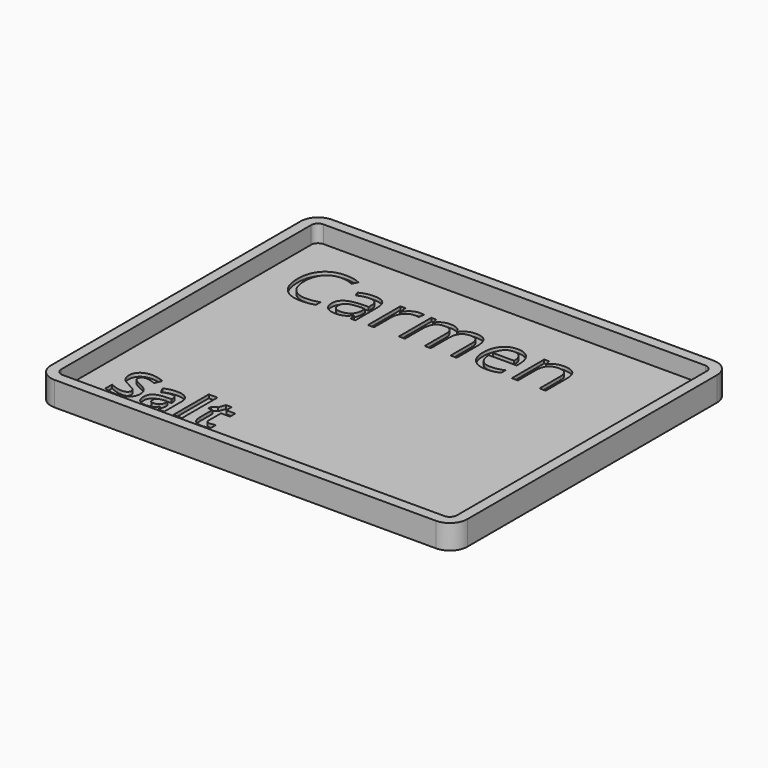
from build123d import *

# Parameters (mm, degrees)
F0_W         = 120
F0_H         = 100
F1_DEPTH     = 2
F2_W         = 120
F2_H         = 100
F2_W_2       = 114
F2_H_2       = 94
F3_DEPTH     = 5
F4_R         = 5
F5_R         = 2
F7_TEXT_SIZE = 16.8295455322
F8_DEPTH     = 1
F6_TEXT_SIZE = 21.8341385739
F9_DEPTH     = 1


# Not quite as in the source:
# - Text() gives the source's letters only with a copy of the font that has no kerning and outlines rounded to 1/6400 em; it was checked with that copy


with BuildPart() as f1:
    # F0 (on Top) → F1 (new body)
    with BuildSketch(Plane.XY):
        Rectangle(F0_W, F0_H)
    extrude(amount=F1_DEPTH)

    # F2 (on face) → F3 (join)
    with BuildSketch(Plane.XY.offset(2)):
        Rectangle(F2_W, F2_H)
        Rectangle(F2_W_2, F2_H_2, mode=Mode.SUBTRACT)
    extrude(amount=F3_DEPTH)

    # F4
    f4_edges = [f1.edges().sort_by_distance(p)[0] for p in [
        (-60, -50, 3.5),
        (60, -50, 3.5),
        (60, 50, 3.5),
        (-60, 50, 3.5),
    ]]
    fillet(f4_edges, radius=F4_R)

    # F5
    f5_edges = [f1.edges().sort_by_distance(p)[0] for p in [
        (-57, 47, 4.5),
        (57, 47, 4.5),
        (57, -47, 4.5),
        (-57, -47, 4.5),
    ]]
    fillet(f5_edges, radius=F5_R)

    # F7 (on face) → F8 (cut)
    with BuildSketch(Plane.XY.offset(2)):
        with Locations((-50.1878341356, -39.1101905724)):
            Text('Salt', F7_TEXT_SIZE, font='Open Sans', font_style=FontStyle.BOLD, text_align=(TextAlign.LEFT, TextAlign.BOTTOM))
    extrude(amount=-F8_DEPTH, mode=Mode.SUBTRACT)

    # F6 (on face) → F9 (cut)
    with BuildSketch(Plane.XY.offset(2)):
        with Locations((-50.3781922162, 22.4355906248)):
            Text('Carmen', F6_TEXT_SIZE, font='Open Sans', text_align=(TextAlign.LEFT, TextAlign.BOTTOM))
    extrude(amount=-F9_DEPTH, mode=Mode.SUBTRACT)


solid = f1.part
